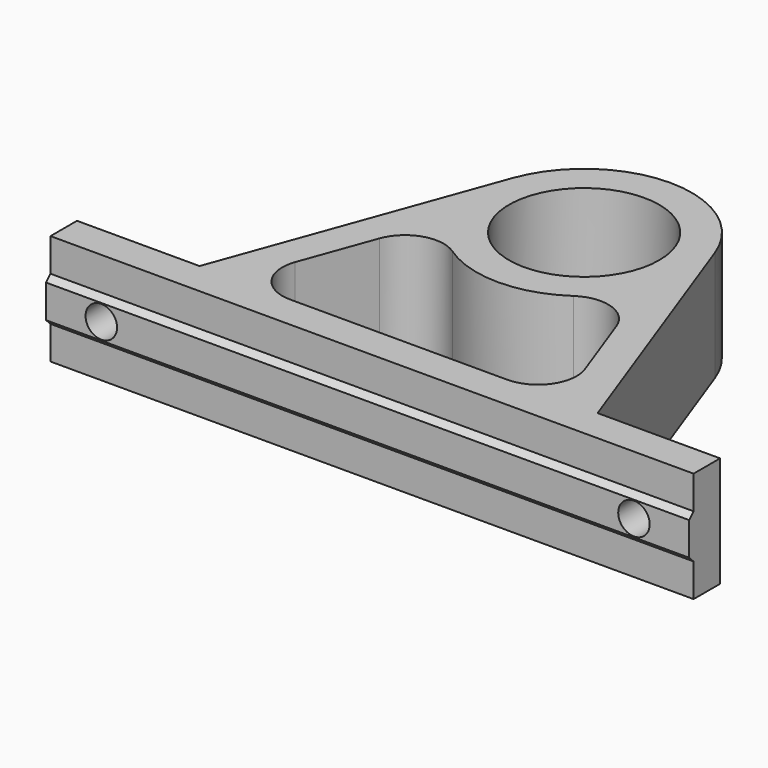
from build123d import *

# Parameters (mm, degrees)
F0_R        = 13.6
F0_W        = 59.3062995352
F0_H        = 6
F1_DEPTH    = 20
F2_R        = 7
F3_W        = 116.4440756161
F3_H        = 2
F4_DEPTH    = 1
F5_T4_DEPTH = 116.4440756161
F5_T9_DEPTH = 116.4440756161
F6_R        = 2.85
F7_DEPTH    = 25


# Not quite as in the source:
# - a fillet or chamfer that OpenCascade refuses, or shapes differently, is made with other operations: its cross-section is extruded or revolved along the edge and cut away or added


with BuildPart() as f1:
    # F0 (on Top) → F1 (new body)
    with BuildSketch(Plane.XY):
        with BuildLine():
            ThreePointArc((17.4985003919, 39.3946247011), (18.9930350082, 43.5824643545), (19.5, 48))
            ThreePointArc((19.5, 48), (19.2037511837, 51.3861394645), (18.3240061053, 54.6693927949))
            ThreePointArc((18.3240061053, 54.6693927949), (0, 67.5), (-18.3240061053, 54.6693927949))
            ThreePointArc((-18.3240061053, 54.6693927949), (-19.4715851439, 46.9476825647), (-17.4985003919, 39.3946247011))
            ThreePointArc((-17.4985003919, 39.3946247011), (0, 28.5), (17.4985003919, 39.3946247011))
        make_face()
        with Locations((0, 48)):
            Circle(F0_R, mode=Mode.SUBTRACT)
        with BuildLine():
            ThreePointArc((-17.4985003919, 39.3946247011), (-19.4715851439, 46.9476825647), (-18.3240061053, 54.6693927949))
            Line((-18.3240061053, 54.6693927949), (-36.0382164025, 6))
            Line((-36.0382164025, 6), (-29.6531497676, 6))
            Line((-29.6531497676, 6), (-17.4985003919, 39.3946247011))
        make_face()
        Polygon((-29.6531497676, 6), (-36.0382164025, 6), (-38.2220378081, 0), (-29.6531497676, 0), align=None)
        Polygon((-38.2220378081, 0), (-36.0382164025, 6), (-58.2220378081, 6), (-58.2220378081, 0), align=None)
        with Locations((0, 3)):
            Rectangle(F0_W, F0_H)
        Polygon((38.2220378081, 0), (36.0382164025, 6), (29.6531497676, 6), (29.6531497676, 0), align=None)
        Polygon((58.2220378081, 6), (36.0382164025, 6), (38.2220378081, 0), (58.2220378081, 0), align=None)
        with BuildLine():
            ThreePointArc((18.3240061053, 54.6693927949), (19.2037511837, 51.3861394645), (19.5, 48))
            ThreePointArc((19.5, 48), (18.9930350082, 43.5824643545), (17.4985003919, 39.3946247011))
            Line((17.4985003919, 39.3946247011), (29.6531497676, 6))
            Line((29.6531497676, 6), (36.0382164025, 6))
            Line((36.0382164025, 6), (18.3240061053, 54.6693927949))
        make_face()
    extrude(amount=F1_DEPTH)

    # F2
    f2_edges = [f1.edges().sort_by_distance(p)[0] for p in [
        (-17.4985, 39.394625, 10),
        (17.4985, 39.394625, 10),
        (-29.65315, 6, 10),
        (29.65315, 6, 10),
    ]]
    fillet(f2_edges, radius=F2_R)

    # F3 (on face) → F4 (join)
    with BuildSketch(Plane.XZ):
        with Locations((0, 10)):
            Rectangle(F3_W, F3_H)
    extrude(amount=F4_DEPTH)

    # F5: chamfer of 3 on 2 edges, made by hand


with BuildPart() as f5_tool2:
    # F5_s3 → F5_t4 (new body)
    with BuildSketch(Plane.YZ.offset(58.2220378081)):
        Polygon((0, 14), (-3, 11), (0, 11), align=None)
    extrude(amount=-F5_T4_DEPTH)

    split(bisect_by=Plane.XZ.offset(1), keep=Keep.BOTTOM)


with BuildPart() as f1_1:
    add(f1.part)

    # F5_t1: union F5_tool2
    add(f5_tool2.part)


with BuildPart() as f5_tool7:
    # F5_s8 → F5_t9 (new body)
    with BuildSketch(Plane.YZ.offset(-58.2220378081)):
        Polygon((0, 6), (-3, 9), (0, 9), align=None)
    extrude(amount=F5_T9_DEPTH)

    split(bisect_by=Plane.XZ.offset(1), keep=Keep.BOTTOM)


with BuildPart() as f1_2:
    add(f1_1.part)

    # F5_t6: union F5_tool7
    add(f5_tool7.part)

    # F6 (on face) → F7 (cut)
    with BuildSketch(Plane(origin=(0, 6, 0), x_dir=(-1, 0, 0), z_dir=(0, 1, 0))):
        with Locations((48.2220378081, 10)):
            Circle(F6_R)
        with Locations((-48.2220378081, 10)):
            Circle(F6_R)
    extrude(amount=-F7_DEPTH, mode=Mode.SUBTRACT)


solid = f1_2.part
